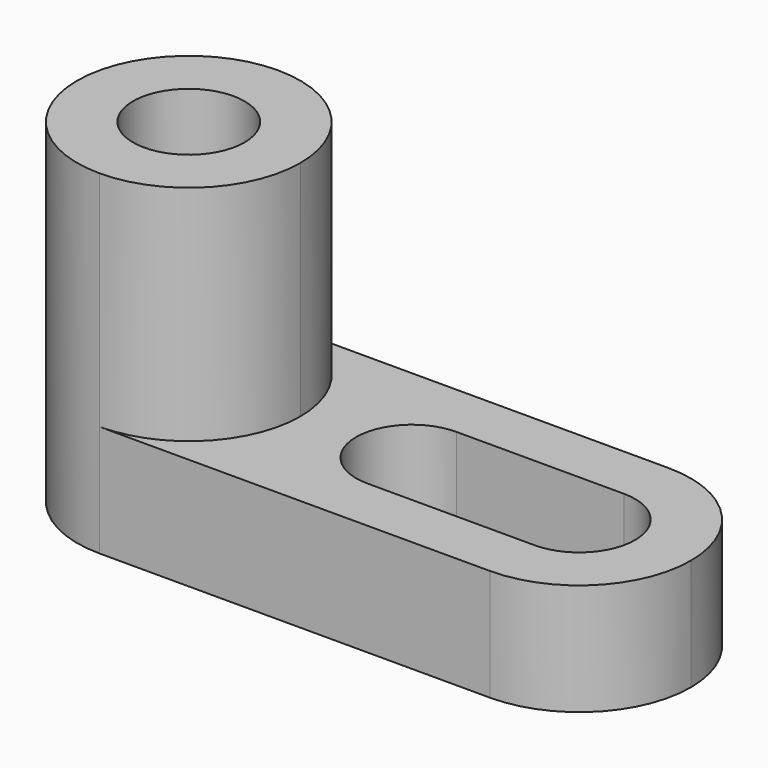
from build123d import *

# Parameters (mm, degrees)
F0_R     = 6.35
F1_DEPTH = 12.7
F2_DEPTH = 38.1
F3_DEPTH = 25.4
F5_DEPTH = 25.4
F7_DEPTH = 25.4


with BuildPart() as f1:
    # F0 (on Top) → F1 (new body)
    with BuildSketch(Plane.XY):
        with BuildLine():
            Line((-42.708286, 25.4), (-42.708286, 12.7))
            ThreePointArc((-42.708286, 12.7), (-38.988542, 21.680256), (-30.008286, 25.4))
            Line((-30.008286, 25.4), (-42.708286, 25.4))
        make_face()
        with BuildLine():
            ThreePointArc((-17.308286, 12.7), (-21.02803, 3.719744), (-30.008286, 0))
            Line((-30.008286, 0), (27.141714, 0))
            Line((27.141714, 0), (27.141714, 25.4))
            Line((27.141714, 25.4), (-30.008286, 25.4))
            ThreePointArc((-30.008286, 25.4), (-21.02803, 21.680256), (-17.308286, 12.7))
        make_face()
        with BuildLine():
            Line((-42.708286, 12.7), (-42.708286, 0))
            Line((-42.708286, 0), (-30.008286, 0))
            ThreePointArc((-30.008286, 0), (-38.988542, 3.719744), (-42.708286, 12.7))
        make_face()
        with BuildLine():
            ThreePointArc((-30.008286, 25.4), (-38.988542, 21.680256), (-42.708286, 12.7))
            ThreePointArc((-42.708286, 12.7), (-38.988542, 3.719744), (-30.008286, 0))
            ThreePointArc((-30.008286, 0), (-21.02803, 3.719744), (-17.308286, 12.7))
            ThreePointArc((-17.308286, 12.7), (-21.02803, 21.680256), (-30.008286, 25.4))
        make_face()
        with Locations((-30.008286, 12.7)):
            Circle(F0_R, mode=Mode.SUBTRACT)
    extrude(amount=F1_DEPTH)

    # F0 (on Top) → F2 (join)
    with BuildSketch(Plane.XY):
        with BuildLine():
            ThreePointArc((-30.008286, 25.4), (-38.988542, 21.680256), (-42.708286, 12.7))
            ThreePointArc((-42.708286, 12.7), (-38.988542, 3.719744), (-30.008286, 0))
            ThreePointArc((-30.008286, 0), (-21.02803, 3.719744), (-17.308286, 12.7))
            ThreePointArc((-17.308286, 12.7), (-21.02803, 21.680256), (-30.008286, 25.4))
        make_face()
        with Locations((-30.008286, 12.7)):
            Circle(F0_R, mode=Mode.SUBTRACT)
    extrude(amount=F2_DEPTH)

    # F3 (cut): faces of the model
    f3_faces = [f1.faces().sort_by_distance(p)[0] for p in [
        (-39.871513, 22.563227, 12.7),
        (-39.871513, 2.836773, 12.7),
    ]]
    extrude(f3_faces, amount=-F3_DEPTH, mode=Mode.SUBTRACT)

    # F4 (on face) → F5 (cut)
    with BuildSketch(Plane.XY.offset(12.7)):
        with BuildLine():
            ThreePointArc((-4.608286, 19.05), (-0.118158, 17.190128), (1.741714, 12.7))
            ThreePointArc((1.741714, 12.7), (-0.118158, 8.209872), (-4.608286, 6.35))
            Line((-4.608286, 6.35), (14.441714, 6.35))
            ThreePointArc((14.441714, 6.35), (8.091714, 12.7), (14.441714, 19.05))
            Line((14.441714, 19.05), (-4.608286, 19.05))
        make_face()
        with BuildLine():
            ThreePointArc((-4.608286, 6.35), (-0.118158, 8.209872), (1.741714, 12.7))
            ThreePointArc((1.741714, 12.7), (-0.118158, 17.190128), (-4.608286, 19.05))
            Line((-4.608286, 19.05), (-4.608286, 12.7))
            Line((-4.608286, 12.7), (-4.608286, 6.35))
        make_face()
        with BuildLine():
            Line((-4.608286, 12.7), (-4.608286, 19.05))
            ThreePointArc((-4.608286, 19.05), (-10.958286, 12.7), (-4.608286, 6.35))
            Line((-4.608286, 6.35), (-4.608286, 12.7))
        make_face()
        with BuildLine():
            Line((14.441714, 12.7), (14.441714, 19.05))
            ThreePointArc((14.441714, 19.05), (8.091714, 12.7), (14.441714, 6.35))
            Line((14.441714, 6.35), (14.441714, 12.7))
        make_face()
        with BuildLine():
            ThreePointArc((20.791714, 12.7), (18.931842, 17.190128), (14.441714, 19.05))
            Line((14.441714, 19.05), (14.441714, 12.7))
            Line((14.441714, 12.7), (14.441714, 6.35))
            ThreePointArc((14.441714, 6.35), (18.931842, 8.209872), (20.791714, 12.7))
        make_face()
    extrude(amount=-F5_DEPTH, mode=Mode.SUBTRACT)

    # F6 (on face) → F7 (cut)
    with BuildSketch(Plane.XY.offset(12.7)):
        with BuildLine():
            ThreePointArc((14.441714, 25.4), (23.42197, 21.680256), (27.141714, 12.7))
            Line((27.141714, 12.7), (27.141714, 25.4))
            Line((27.141714, 25.4), (14.441714, 25.4))
        make_face()
        with BuildLine():
            Line((27.141714, 0), (27.141714, 12.7))
            ThreePointArc((27.141714, 12.7), (23.42197, 3.719744), (14.441714, 0))
            Line((14.441714, 0), (27.141714, 0))
        make_face()
    extrude(amount=-F7_DEPTH, mode=Mode.SUBTRACT)


solid = f1.part
